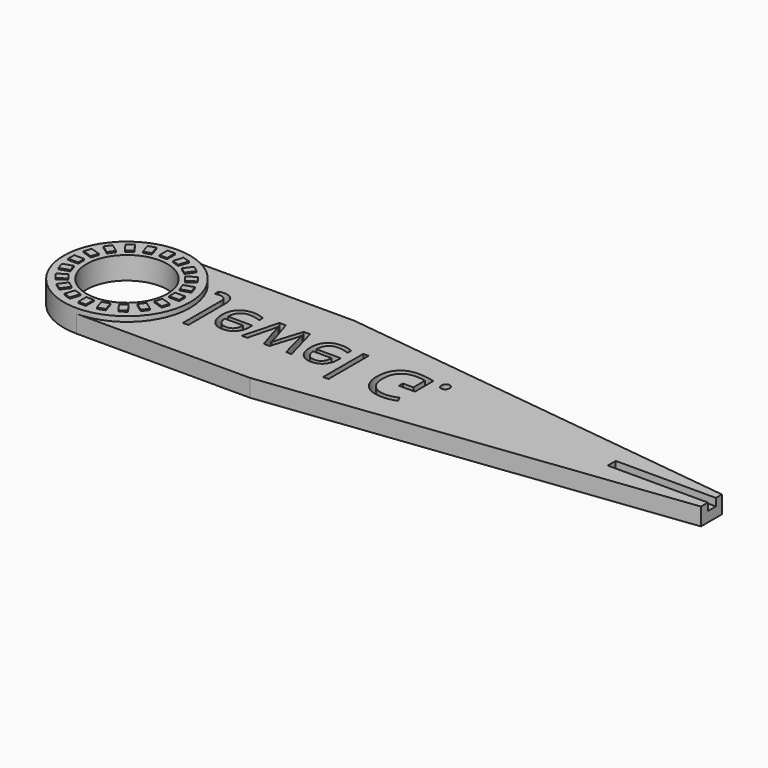
from build123d import *

# Parameters (mm, degrees)
F0_R         = 8.0699934722
F1_DEPTH     = 3.5
F2_R         = 12.6093648002
F2_R_2       = 8.0699934722
F3_DEPTH     = 1
F4_W         = 1.5
F4_H         = 2
F4_W_2       = 2
F4_H_2       = 1.5
F5_DEPTH     = 0.25
F6_W         = 20
F6_H         = 2
F7_DEPTH     = 1.5
F9_TEXT_SIZE = 13.1841955913
F10_DEPTH    = 4.751


# Not quite as in the source:
# - Text() gives the source's letters only with a copy of the font that has no kerning and outlines rounded to 1/6400 em; it was checked with that copy


with BuildPart() as f1:
    # F0 (on Top) → F1 (new body)
    with BuildSketch(Plane.XY):
        with BuildLine():
            Line((35.3062214407, 12.6093648002), (0, 12.6093648002))
            ThreePointArc((0, 12.6093648002), (-12.6093648002, 0), (0, -12.6093648002))
            Line((0, -12.6093648002), (34.6995617834, -12.6093648002))
            Line((34.6995617834, -12.6093648002), (116.6950058753, -2.616078641))
            Line((116.6950058753, -2.616078641), (116.6950058753, 2.616078641))
            Line((116.6950058753, 2.616078641), (35.3062214407, 12.6093648002))
        make_face()
        Circle(F0_R, mode=Mode.SUBTRACT)
    extrude(amount=F1_DEPTH)

    # F2 (on face) → F3 (join)
    with BuildSketch(Plane.XY.offset(3.5)):
        Circle(F2_R)
        Circle(F2_R_2, mode=Mode.SUBTRACT)
    extrude(amount=F3_DEPTH)

    # F4 (on face) → F5 (join)
    with BuildSketch(Plane.XY.offset(4.5)):
        with Locations((0, 10.0699934722)):
            Rectangle(F4_W, F4_H)
        Polygon((-2.7183706851, 10.7678329519), (-4.1449554595, 10.3043074603), (-3.5269214708, 8.4021944277), (-2.1003366963, 8.8657199193), align=None)
        Polygon((-5.9236144903, 9.4086757356), (-7.1371399818, 8.5269978571), (-5.9615694773, 6.9089638684), (-4.7480439857, 7.7906417468), align=None)
        Polygon((-8.5519798197, 7.1255656015), (-9.4336576981, 5.9120401099), (-7.8156237093, 4.7364696053), (-6.9339458309, 5.9499950969), align=None)
        Polygon((-10.3461839619, 4.1419892768), (-10.8097094535, 2.7154045023), (-8.9075964209, 2.0973705136), (-8.4440709293, 3.523955288), align=None)
        with Locations((-10.1305977146, 0)):
            Rectangle(F4_W_2, F4_H_2)
        Polygon((-10.8284371943, -2.7183706851), (-10.3649117027, -4.1449554595), (-8.4627986701, -3.5269214708), (-8.9263241617, -2.1003366963), align=None)
        Polygon((-9.469279978, -5.9236144903), (-8.5876020996, -7.1371399818), (-6.9695681108, -5.9615694773), (-7.8512459893, -4.7480439857), align=None)
        Polygon((-7.1861698439, -8.5519798197), (-5.9726443523, -9.4336576981), (-4.7970738477, -7.8156237093), (-6.0105993393, -6.9339458309), align=None)
        Polygon((-4.2025935192, -10.3461839619), (-2.7760087448, -10.8097094535), (-2.157974756, -8.9075964209), (-3.5845595305, -8.4440709293), align=None)
        with Locations((-0.0606042424, -10.1305977146)):
            Rectangle(F4_W, F4_H)
        Polygon((2.6577664427, -10.8284371943), (4.0843512171, -10.3649117027), (3.4663172284, -8.4627986701), (2.0397324539, -8.9263241617), align=None)
        Polygon((5.8630102478, -9.469279978), (7.0765357394, -8.5876020996), (5.9009652348, -6.9695681108), (4.6874397433, -7.8512459893), align=None)
        Polygon((8.4913755772, -7.1861698439), (9.3730534557, -5.9726443523), (7.7550194669, -4.7970738477), (6.8733415885, -6.0105993393), align=None)
        Polygon((10.2855797195, -4.2025935192), (10.749105211, -2.7760087448), (8.8469921784, -2.157974756), (8.3834666869, -3.5845595305), align=None)
        with Locations((10.0699934722, -0.0606042424)):
            Rectangle(F4_W_2, F4_H_2)
        Polygon((10.7678329519, 2.6577664427), (10.3043074603, 4.0843512171), (8.4021944277, 3.4663172284), (8.8657199193, 2.0397324539), align=None)
        Polygon((9.4086757356, 5.8630102478), (8.5269978571, 7.0765357394), (6.9089638684, 5.9009652348), (7.7906417468, 4.6874397433), align=None)
        Polygon((7.1255656015, 8.4913755772), (5.9120401099, 9.3730534557), (4.7364696053, 7.7550194669), (5.9499950969, 6.8733415885), align=None)
        Polygon((4.1419892768, 10.2855797195), (2.7154045023, 10.749105211), (2.0973705136, 8.8469921784), (3.523955288, 8.3834666869), align=None)
    extrude(amount=F5_DEPTH)

    # F6 (on face) → F7 (cut)
    with BuildSketch(Plane.XY.offset(3.5)):
        with Locations((106.6950058753, 0.116078641)):
            Rectangle(F6_W, F6_H)
    extrude(amount=-F7_DEPTH, mode=Mode.SUBTRACT)

    # F9 (on face) → F10 (cut, through all)
    with BuildSketch(Plane(origin=(0, 0, 0), x_dir=(1, 0, 0), z_dir=(0, 0, -1))):
        with Locations((13.67960684, -4.7463104129)):
            Text('Jewel G.', F9_TEXT_SIZE, font='Open Sans', text_align=(TextAlign.LEFT, TextAlign.BOTTOM))
    extrude(amount=-F10_DEPTH, mode=Mode.SUBTRACT)


solid = f1.part
